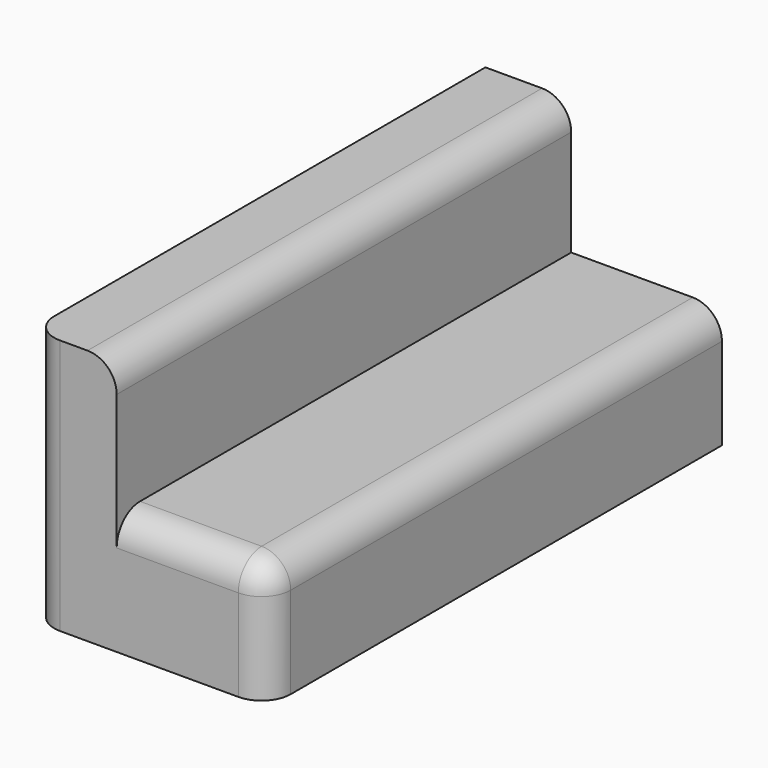
from build123d import *

# Parameters (mm, degrees)
F1_DEPTH    = 1981.2
F2_R        = 101.6
F3_R        = 101.6
F4_T1_DEPTH = 2133.6
F4_S5_W     = 101.6
F4_S5_H     = 101.6
F4_T6_DEPTH = 101.6


# Not quite as in the source:
# - a fillet or chamfer that OpenCascade refuses, or shapes differently, is made with other operations: its cross-section is extruded or revolved along the edge and cut away or added


with BuildPart() as f1:
    # F0 (on Front) → F1 (new body)
    with BuildSketch(Plane.XZ):
        Polygon((251.7913877964, 36.7387868464), (-47.3107099533, 36.7387868464), (-47.3107099533, -855.4236292839), (777.5030732155, -855.4236292839), (777.5030732155, -434.3872666359), (251.7913877964, -434.3872666359), align=None)
    extrude(amount=F1_DEPTH)

    # F2
    f2_edges = [f1.edges().sort_by_distance(p)[0] for p in [
        (251.791388, -990.6, 36.738787),
        (-47.31071, -1981.2, -409.342421),
    ]]
    fillet(f2_edges, radius=F2_R)

    # F3
    f3_edges = [f1.edges().sort_by_distance(p)[0] for p in [
        (514.647231, -1981.2, -434.387267),
        (777.503073, -1981.2, -644.905448),
    ]]
    fillet(f3_edges, radius=F3_R)

    # F4: fillet of radius 101.6 on 1 edges, made by hand

    # F4_s2 → F4_t1 (cut)
    with BuildSketch(Plane.XZ.offset(-254)):
        with BuildLine():
            ThreePointArc((777.5030732155, -535.9872666359), (747.745122184, -464.1452176673), (675.9030732155, -434.3872666359))
            Line((675.9030732155, -434.3872666359), (777.5030732155, -434.3872666359))
            Line((777.5030732155, -434.3872666359), (777.5030732155, -535.9872666359))
        make_face()
    extrude(amount=F4_T1_DEPTH, mode=Mode.SUBTRACT)


with BuildPart() as f4_tool4:
    # F4_s5 → F4_t6 (new body)
    with BuildSketch(Plane.YZ.offset(675.9030732155)):
        with Locations((-1930.4, -485.1872666359)):
            Rectangle(F4_S5_W, F4_S5_H)
    extrude(amount=F4_T6_DEPTH)

    # F4_s7 → F4_t8 (revolve, cut)
    with BuildSketch(Plane(origin=(675.9030732155, -1879.6, -535.9872666359), x_dir=(0, 0.7071067812, -0.7071067812), z_dir=(0, -0.7071067812, -0.7071067812))):
        with BuildLine():
            ThreePointArc((0, -101.6), (101.6, 0), (0, 101.6))
            Line((0, 101.6), (0, -101.6))
        make_face()
    revolve(axis=Axis((675.9030732155, -1879.6, -535.9872666359), (1, 0, 0)), mode=Mode.SUBTRACT)


with BuildPart() as f1_1:
    add(f1.part)

    # F4_t3: cut F4_tool4
    add(f4_tool4.part, mode=Mode.SUBTRACT)


solid = f1_1.part
